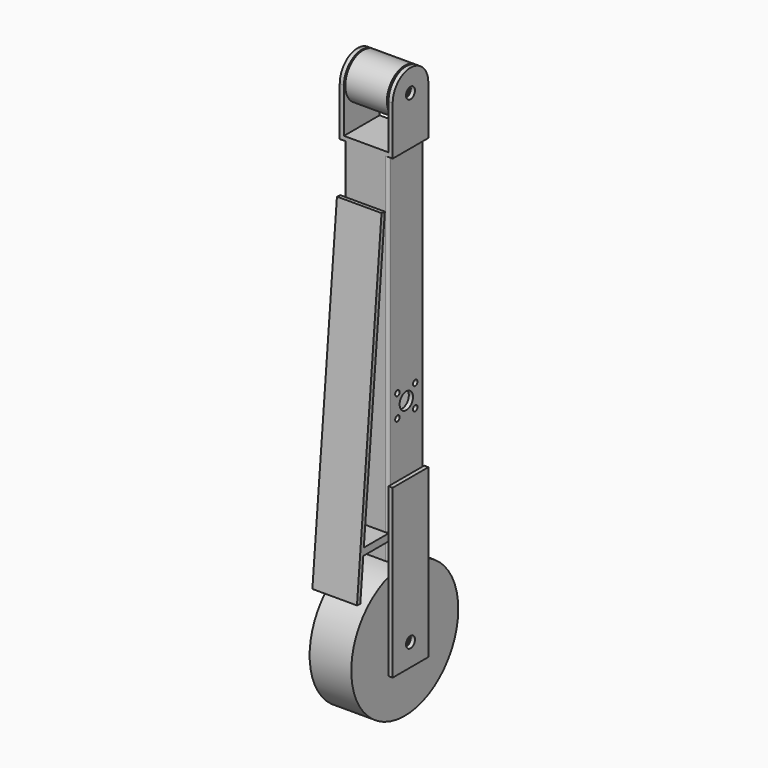
from build123d import *

# Parameters (mm, degrees)
F1_DEPTH       = 406.4
F2_W           = 60.325
F2_H           = 50.8
F3_DEPTH       = 4.7625
F4_W           = 4.7625
F4_H           = 50.8
F5_DEPTH       = 76.2
F6_R           = 6.35
F7_DEPTH       = 60.326
F9_DEPTH       = 4.7625
F10_W          = 50.8
F10_H          = 190.5
F11_DEPTH      = 4.7625
F12_W          = 50.8
F12_H          = 190.5
F13_DEPTH      = 4.7625
F14_R          = 6.35
F15_DEPTH      = 60.326
F17_DEPTH      = 60.326
F19_START      = 1.5875
F18_R          = 6.35
F19_DEPTH      = 47.4345
F21_START      = 1.5875
F20_R          = 76.2
F20_R_2        = 6.35
F21_DEPTH      = 47.4345
F23_DEPTH      = 25.4
F23_DEPTH_BACK = 25.4
F24_R          = 9.525
F25_DEPTH      = 55.5635


with BuildPart() as f1:
    # F0 (on Top) → F1 (new body)
    with BuildSketch(Plane.XY):
        with BuildLine():
            ThreePointArc((25.4, 22.225), (24.4700640303, 24.4700640303), (22.225, 25.4))
            Line((22.225, 25.4), (-22.225, 25.4))
            ThreePointArc((-22.225, 25.4), (-24.4700640303, 24.4700640303), (-25.4, 22.225))
            Line((-25.4, 22.225), (-25.4, -22.225))
            ThreePointArc((-25.4, -22.225), (-24.4700640303, -24.4700640303), (-22.225, -25.4))
            Line((-22.225, -25.4), (22.225, -25.4))
            ThreePointArc((22.225, -25.4), (24.4700640303, -24.4700640303), (25.4, -22.225))
            Line((25.4, -22.225), (25.4, 22.225))
        make_face()
        with BuildLine():
            Line((-17.4625, 20.6375), (17.4625, 20.6375))
            ThreePointArc((17.4625, 20.6375), (19.7075640303, 19.7075640303), (20.6375, 17.4625))
            Line((20.6375, 17.4625), (20.6375, -17.4625))
            ThreePointArc((20.6375, -17.4625), (19.7075640303, -19.7075640303), (17.4625, -20.6375))
            Line((17.4625, -20.6375), (-17.4625, -20.6375))
            ThreePointArc((-17.4625, -20.6375), (-19.7075640303, -19.7075640303), (-20.6375, -17.4625))
            Line((-20.6375, -17.4625), (-20.6375, 17.4625))
            ThreePointArc((-20.6375, 17.4625), (-19.7075640303, 19.7075640303), (-17.4625, 20.6375))
        make_face(mode=Mode.SUBTRACT)
    extrude(amount=F1_DEPTH)

    # F2 (on face) → F3 (join)
    with BuildSketch(Plane.XY.offset(406.4)):
        Rectangle(F2_W, F2_H)
    extrude(amount=F3_DEPTH)

    # F4 (on face) → F5 (join)
    with BuildSketch(Plane.XY.offset(411.1625)):
        with Locations((-27.78125, 0)):
            Rectangle(F4_W, F4_H)
        with Locations((27.78125, 0)):
            Rectangle(F4_W, F4_H)
    extrude(amount=F5_DEPTH)

    # F6 (on face) → F7 (cut, through all)
    with BuildSketch(Plane.YZ.offset(30.1625)):
        with Locations((0, 461.9625)):
            Circle(F6_R)
    extrude(amount=-F7_DEPTH, mode=Mode.SUBTRACT)

    # F8 (on Top) → F9 (join)
    with BuildSketch(Plane.XY):
        with BuildLine():
            Line((-22.225, -25.4), (22.225, -25.4))
            ThreePointArc((22.225, -25.4), (24.4700640303, -24.4700640303), (25.4, -22.225))
            Line((25.4, -22.225), (25.4, 22.225))
            ThreePointArc((25.4, 22.225), (24.4700640303, 24.4700640303), (22.225, 25.4))
            Line((22.225, 25.4), (-22.225, 25.4))
            ThreePointArc((-22.225, 25.4), (-24.4700640303, 24.4700640303), (-25.4, 22.225))
            Line((-25.4, 22.225), (-25.4, -22.225))
            ThreePointArc((-25.4, -22.225), (-24.4700640303, -24.4700640303), (-22.225, -25.4))
        make_face()
    extrude(amount=F9_DEPTH)

    # F10 (on face) → F11 (join)
    with BuildSketch(Plane.YZ.offset(25.4)):
        with Locations((0, -19.05)):
            Rectangle(F10_W, F10_H)
    extrude(amount=F11_DEPTH)

    # F12 (on face) → F13 (join)
    with BuildSketch(Plane(origin=(-25.4, 0, 0), x_dir=(0, -1, 0), z_dir=(-1, 0, 0))):
        with Locations((0, -19.05)):
            Rectangle(F12_W, F12_H)
    extrude(amount=F13_DEPTH)

    # F14 (on face) → F15 (cut, through all)
    with BuildSketch(Plane.YZ.offset(30.1625)):
        with Locations((0, -88.9)):
            Circle(F14_R)
    extrude(amount=-F15_DEPTH, mode=Mode.SUBTRACT)

    # F16 (on face) → F17 (cut, through all)
    with BuildSketch(Plane.YZ.offset(30.1625)):
        with BuildLine():
            ThreePointArc((0, 487.3625000002), (17.9605122422, 479.9230122422), (25.4000000002, 461.9625))
            Line((25.4, 461.9625), (25.4, 487.3625))
            Line((25.4, 487.3625), (0, 487.3625))
        make_face()
        with BuildLine():
            Line((-25.4, 487.3625), (-25.4, 461.9625))
            ThreePointArc((-25.4000000002, 461.9625), (-17.9605122422, 479.9230122422), (0, 487.3625000002))
            Line((0, 487.3625), (-25.4, 487.3625))
        make_face()
    extrude(amount=-F17_DEPTH, mode=Mode.SUBTRACT)

    # F22 (on Right) → F23 (join, two sides)
    with BuildSketch(Plane.YZ) as f23_sk:
        Polygon((-35.3324371131, 354.2576350563), (-70.3194279932, -25.132547301), (-65.5770507137, -25.569884687), (-61.2947668437, 20.8661310292), (-60.5542488364, 28.896123171), (-30.5900598336, 353.8202976703), align=None)
        Polygon((-60.5542488364, 28.896123171), (-61.2947668437, 20.8661310292), (-23.283880204, 20.8661310292), (-23.283880204, 28.896123171), align=None)
    extrude(amount=F23_DEPTH)
    extrude(f23_sk.sketch, amount=-F23_DEPTH_BACK)

    # F24 (on face) → F25 (cut, through all)
    with BuildSketch(Plane.YZ.offset(25.4)):
        with Locations((0, 151.7015000002)):
            Circle(F24_R)
        with BuildLine():
            Line((12.7, 161.2265000002), (12.7, 164.4015000002))
            Line((12.7, 164.4015000002), (9.525, 164.4015000002))
            ThreePointArc((9.525, 164.4015000002), (10.4549359697, 162.1564359699), (12.7, 161.2265000002))
        make_face()
        with BuildLine():
            Line((9.525, 164.4015000002), (12.7, 164.4015000002))
            Line((12.7, 164.4015000002), (12.7, 161.2265000002))
            ThreePointArc((12.7, 161.2265000002), (14.9450640303, 162.1564359699), (15.875, 164.4015000002))
            ThreePointArc((15.875, 164.4015000002), (12.7, 167.5765000002), (9.525, 164.4015000002))
        make_face()
        with BuildLine():
            Line((12.7, 142.1765000002), (12.7, 139.0015000002))
            Line((12.7, 139.0015000002), (9.525, 139.0015000002))
            ThreePointArc((9.525, 139.0015000002), (12.7, 135.8265000002), (15.875, 139.0015000002))
            ThreePointArc((15.875, 139.0015000002), (14.9450640303, 141.2465640304), (12.7, 142.1765000002))
        make_face()
        with BuildLine():
            Line((9.525, 139.0015000002), (12.7, 139.0015000002))
            Line((12.7, 139.0015000002), (12.7, 142.1765000002))
            ThreePointArc((12.7, 142.1765000002), (10.4549359697, 141.2465640304), (9.525, 139.0015000002))
        make_face()
        with BuildLine():
            Line((-9.525, 164.4015000002), (-12.7, 164.4015000002))
            Line((-12.7, 164.4015000002), (-12.7, 161.2265000002))
            ThreePointArc((-12.7, 161.2265000002), (-10.4549359697, 162.1564359699), (-9.525, 164.4015000002))
        make_face()
        with BuildLine():
            Line((-12.7, 161.2265000002), (-12.7, 164.4015000002))
            Line((-12.7, 164.4015000002), (-9.525, 164.4015000002))
            ThreePointArc((-9.525, 164.4015000002), (-14.9450640303, 166.6465640304), (-12.7, 161.2265000002))
        make_face()
        with BuildLine():
            Line((-12.7, 139.0015000002), (-9.525, 139.0015000002))
            ThreePointArc((-9.525, 139.0015000002), (-10.4549359697, 141.2465640304), (-12.7, 142.1765000002))
            Line((-12.7, 142.1765000002), (-12.7, 139.0015000002))
        make_face()
        with BuildLine():
            ThreePointArc((-12.7, 142.1765000002), (-14.9450640303, 136.7564359699), (-9.525, 139.0015000002))
            Line((-9.525, 139.0015000002), (-12.7, 139.0015000002))
            Line((-12.7, 139.0015000002), (-12.7, 142.1765000002))
        make_face()
    extrude(amount=-F25_DEPTH, mode=Mode.SUBTRACT)


with BuildPart() as f19:
    # F18 (on face) → F19 (new body)
    with BuildSketch(Plane.YZ.offset(-25.4).offset(F19_START)):
        with BuildLine():
            ThreePointArc((-25.4, 461.9625), (0, 436.5625), (25.4, 461.9625))
            ThreePointArc((25.4, 461.9625), (0, 487.3625), (-25.4, 461.9625))
        make_face()
        with Locations((0, 461.9625)):
            Circle(F18_R, mode=Mode.SUBTRACT)
    extrude(amount=F19_DEPTH)


with BuildPart() as f21:
    # F20 (on face) → F21 (new body)
    with BuildSketch(Plane.YZ.offset(-25.4).offset(F21_START)):
        with Locations((0, -88.9)):
            Circle(F20_R)
        with Locations((0, -88.9)):
            Circle(F20_R_2, mode=Mode.SUBTRACT)
    extrude(amount=F21_DEPTH)


solid = Compound([f1.part, f19.part, f21.part])
